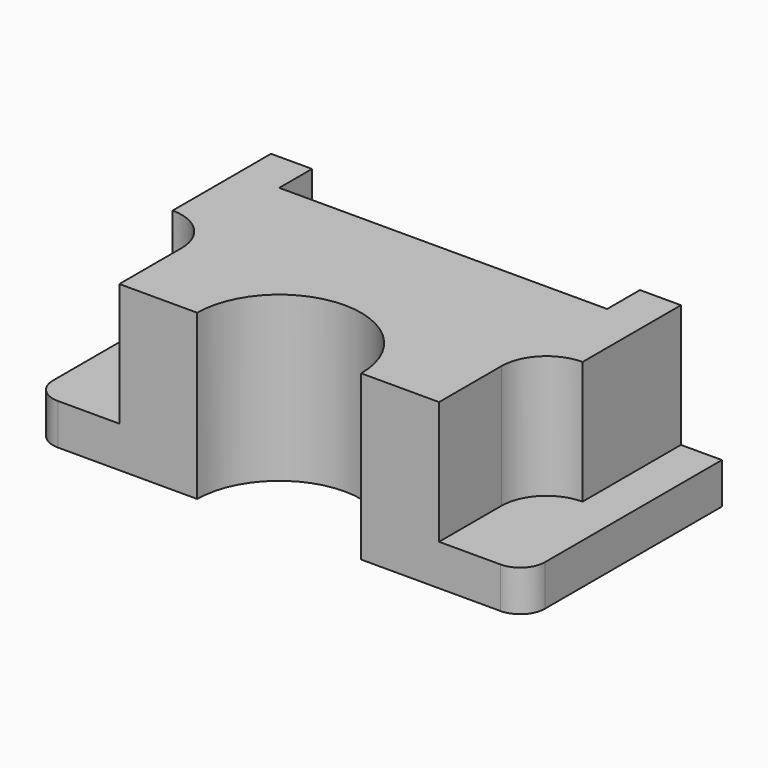
from build123d import *

# Parameters (mm, degrees)
F0_W      = 76.2
F0_H      = 38.1
F1_DEPTH  = 25.4
F2_W      = 50.8
F2_H      = 6.35
F3_DEPTH  = 19.05
F4_W      = 6.35
F4_H      = 38.1
F5_DEPTH  = 19.05
F7_DEPTH  = 25.4
F8_R      = 3.81
F9_W      = 6.985
F9_H      = 19.05
F9_W_2    = 6.9872894436
F10_DEPTH = 19.05
F11_R     = 6.98499


# Not quite as in the source:
# - a fillet or chamfer is up to 0.001 mm smaller than in the source, because OpenCascade refuses the exact size
# - a feature of the source that left no trace in its solid (it failed there, or was rolled back) is left out


with BuildPart() as f1:
    # F0 (on Top) → F1 (new body)
    with BuildSketch(Plane.XY):
        Rectangle(F0_W, F0_H)
    extrude(amount=F1_DEPTH)

    # F2 (on face) → F3 (cut)
    with BuildSketch(Plane.XY.offset(25.4)):
        with Locations((0, 15.875)):
            Rectangle(F2_W, F2_H)
    extrude(amount=-F3_DEPTH, mode=Mode.SUBTRACT)

    # F4 (on face) → F5 (cut)
    with BuildSketch(Plane.XY.offset(25.4)):
        with Locations((-34.925, 0)):
            Rectangle(F4_W, F4_H)
        with Locations((34.925, 0)):
            Rectangle(F4_W, F4_H)
    extrude(amount=-F5_DEPTH, mode=Mode.SUBTRACT)

    # F6 (on face) → F7 (cut)
    with BuildSketch(Plane.XY.offset(25.4)):
        with BuildLine():
            Line((-12.7, -19.05), (12.7, -19.05))
            ThreePointArc((12.7, -19.05), (0, -6.35), (-12.7, -19.05))
        make_face()
    extrude(amount=-F7_DEPTH, mode=Mode.SUBTRACT)

    # F8
    f8_edges = [f1.edges().sort_by_distance(p)[0] for p in [
        (38.1, -19.05, 3.175),
        (-38.1, -19.05, 3.175),
    ]]
    fillet(f8_edges, radius=F8_R)

    # F9 (on face) → F10 (cut)
    with BuildSketch(Plane.XY.offset(25.4)):
        with Locations((-28.2575, -9.525)):
            Rectangle(F9_W, F9_H)
        with Locations((28.2563552782, -9.525)):
            Rectangle(F9_W_2, F9_H)
    extrude(amount=-F10_DEPTH, mode=Mode.SUBTRACT)

    # F11 (radius 6.985 in the source; OpenCascade refuses exactly that, so slightly less here)
    f11_edges = [f1.edges().sort_by_distance(p)[0] for p in [
        (24.762711, 0, 15.875),
        (-24.765, 0, 15.875),
    ]]
    fillet(f11_edges, radius=F11_R)


solid = f1.part
